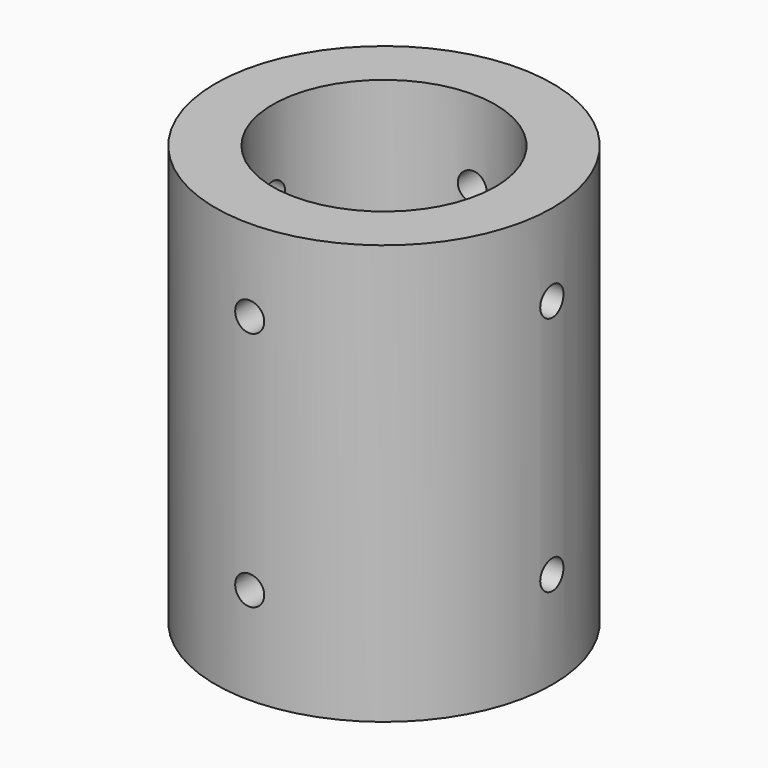
from build123d import *

# Parameters (mm, degrees)
F2_R            = 2.25
F3_DEPTH        = 28
F3_COPIES_COUNT = 4


# Not quite as in the source:
# - a pattern or mirror of a feature is missing from the dataset's text; its kind, count and spacing are read off the source's solid


with BuildPart() as f1:
    # F0 (on Front) → F1 (revolve)
    with BuildSketch(Plane.XZ):
        Polygon((26.1, 27.5), (17.25, 27.5), (17.25, 2.5), (17.25, -2.5), (21.1, -2.5), (21.1, -37.5), (26.1, -37.5), align=None)
    revolve(axis=Axis((0, 0, 0), (0, 0, -1)))

    # F2 (on Front) → F3 (cut)
    with BuildSketch(Plane.XZ):
        with Locations((0, 14.8)):
            Circle(F2_R)
        with Locations((0, -22.5)):
            Circle(F2_R)
    f3 = extrude(amount=-F3_DEPTH, mode=Mode.SUBTRACT)

    # F3_copies: F3 ×4 about axis
    f3_copies_axis = Axis((0, 0, 0), (0, 0, 1))
    for i in range(1, F3_COPIES_COUNT):
        add(f3.rotate(f3_copies_axis, i * 360 / F3_COPIES_COUNT), mode=Mode.SUBTRACT)


solid = f1.part
